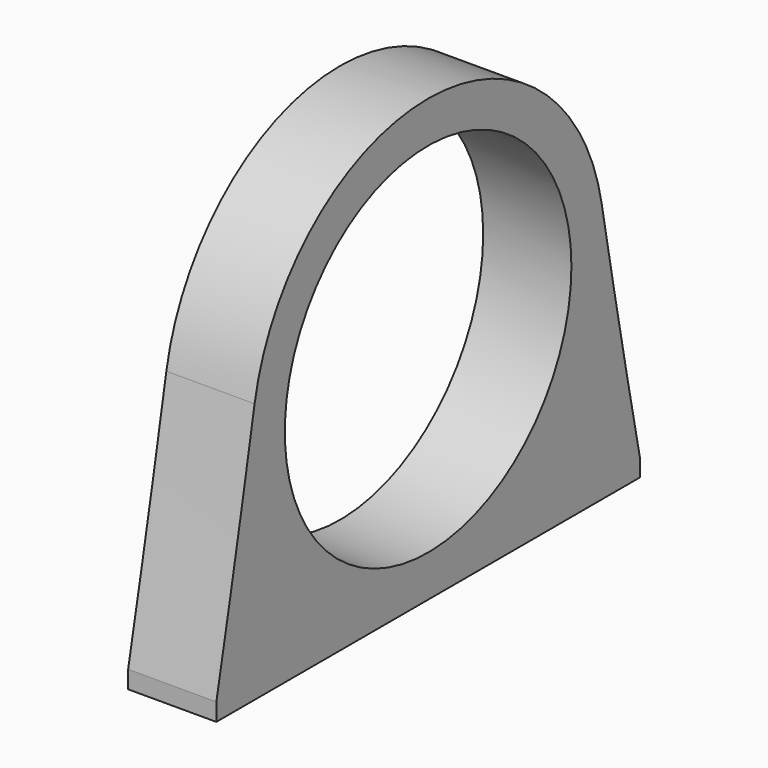
from build123d import *

# Parameters (mm, degrees)
F0_R        = 10.15
F0_W        = 30
F0_H        = 1
F1_DEPTH    = 5
F2_T1_DEPTH = 5
F3_R        = 1.45
F4_DEPTH    = 6


# Not quite as in the source:
# - a fillet or chamfer that OpenCascade refuses, or shapes differently, is made with other operations: its cross-section is extruded or revolved along the edge and cut away or added


with BuildPart() as f1:
    # F0 (on Right) → F1 (new body)
    with BuildSketch(Plane.YZ):
        with BuildLine():
            Line((15, -11.5), (12.5, 0))
            ThreePointArc((12.5, 0), (0, 12.5), (-12.5, 0))
            Line((-12.5, 0), (-15, -11.5))
            Line((-15, -11.5), (15, -11.5))
        make_face()
        Circle(F0_R, mode=Mode.SUBTRACT)
        with Locations((0, -12)):
            Rectangle(F0_W, F0_H)
    extrude(amount=F1_DEPTH)

    # F2: fillet of radius 608.1441737805 on 2 edges, made by hand

    # F2_s2 → F2_t1 (join)
    with BuildSketch(Plane.YZ):
        with BuildLine():
            ThreePointArc((-15, -11.5), (-13.6063343728, -4.6226980795), (-12.2921141837, 2.2702266177))
            ThreePointArc((-12.2921141837, 2.2702266177), (-12.4479200531, 1.1398624268), (-12.5, 0))
            Line((-12.5, 0), (-15, -11.5))
        make_face()
        with BuildLine():
            ThreePointArc((15, -11.5), (13.6063343728, -4.6226980795), (12.2921141837, 2.2702266177))
            ThreePointArc((12.2921141837, 2.2702266177), (12.4479200531, 1.1398624268), (12.5, 0))
            Line((12.5, 0), (15, -11.5))
        make_face()
    extrude(amount=F2_T1_DEPTH)

    # F3 (on face) → F4 (cut)
    with BuildSketch(Plane(origin=(0, 0, -12.5), x_dir=(1, 0, 0), z_dir=(0, 0, -1))):
        with Locations((2.4999999441, 11.0743809491)):
            Circle(F3_R)
        with Locations((2.5, -10.09248567)):
            Circle(F3_R)
    extrude(amount=-F4_DEPTH, mode=Mode.SUBTRACT)


solid = f1.part
